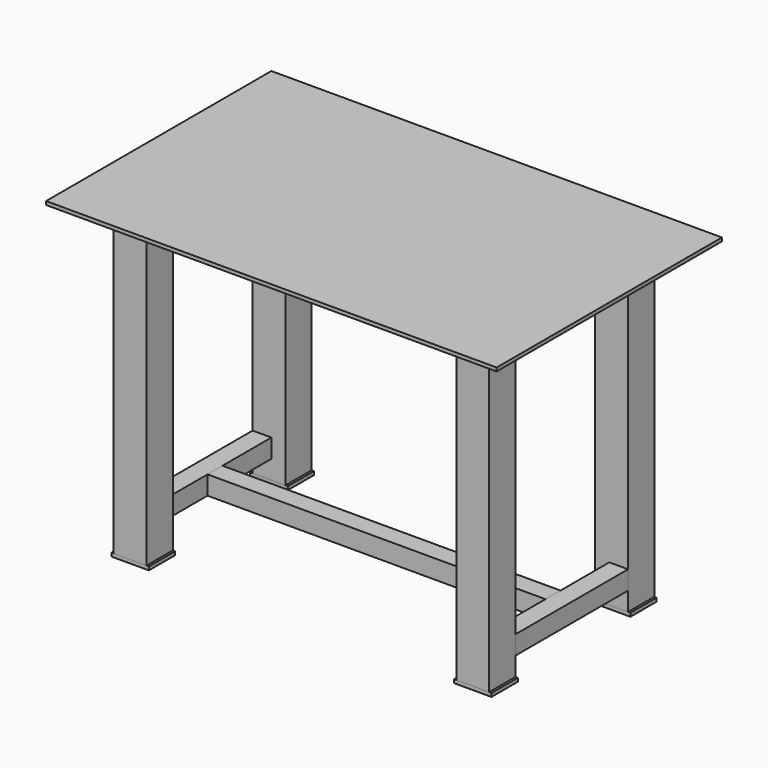
from build123d import *

# Parameters (mm, degrees)
F0_W           = 88.9
F0_H           = 88.9
F0_W_2         = 82.55
F0_H_2         = 82.55
F1_DEPTH       = 838.2
F2_W           = 50.8
F2_H           = 50.8
F2_W_2         = 46.83125
F2_H_2         = 46.83125
F3_DEPTH       = 419.1
F3_DEPTH_BACK  = 419.1
F4_W           = 50.8
F4_H           = 50.8
F4_W_2         = 46.83125
F4_H_2         = 46.83125
F5_DEPTH       = 190.5
F5_DEPTH_BACK  = 190.5
F6_W           = 50.8
F6_H           = 50.8
F6_W_2         = 46.83125
F6_H_2         = 46.83125
F7_DEPTH       = 457.2
F7_DEPTH_BACK  = 457.2
F8_W           = 1219.2
F8_H           = 762
F9_DEPTH       = 9.525
F11_W          = 101.6
F11_H          = 88.9
F12_DEPTH      = 9.525
F15_D          = 7.9375
F15_DEPTH      = 9.525
F15_TIP        = 2.3846655818
F18_W          = 50.8
F18_H          = 50.8
F18_W_2        = 46.83125
F18_H_2        = 46.83125
F19_DEPTH      = 228.6
F19_DEPTH_BACK = 228.6


# Not quite as in the source:
# - a length typed as a fraction of an inch, garbled in the dataset ("3 / 203.2 mm" for 3/8 in), is restored


with BuildPart() as f1:
    # F0 (on Top) → F1 (new body)
    with BuildSketch(Plane.XY):
        with Locations((463.55, -234.95)):
            Rectangle(F0_W, F0_H)
        with Locations((463.55, -234.95)):
            Rectangle(F0_W_2, F0_H_2, mode=Mode.SUBTRACT)
    extrude(amount=-F1_DEPTH)


with BuildPart() as f1b:
    # F0 (on Top) → F1, piece 2 (new body)
    with BuildSketch(Plane.XY):
        with Locations((463.55, 234.95)):
            Rectangle(F0_W, F0_H)
        with Locations((463.55, 234.95)):
            Rectangle(F0_W_2, F0_H_2, mode=Mode.SUBTRACT)
    extrude(amount=-F1_DEPTH)


with BuildPart() as f1c:
    # F0 (on Top) → F1, piece 3 (new body)
    with BuildSketch(Plane.XY):
        with Locations((-463.55, -234.95)):
            Rectangle(F0_W, F0_H)
        with Locations((-463.55, -234.95)):
            Rectangle(F0_W_2, F0_H_2, mode=Mode.SUBTRACT)
    extrude(amount=-F1_DEPTH)


with BuildPart() as f1d:
    # F0 (on Top) → F1, piece 4 (new body)
    with BuildSketch(Plane.XY):
        with Locations((-463.55, 234.95)):
            Rectangle(F0_W, F0_H)
        with Locations((-463.55, 234.95)):
            Rectangle(F0_W_2, F0_H_2, mode=Mode.SUBTRACT)
    extrude(amount=-F1_DEPTH)


with BuildPart() as f3:
    # F2 (on Right) → F3 (new body, two sides)
    with BuildSketch(Plane.YZ) as f3_sk:
        with Locations((-254, -25.4)):
            Rectangle(F2_W, F2_H)
        with Locations((-254, -25.4)):
            Rectangle(F2_W_2, F2_H_2, mode=Mode.SUBTRACT)
    extrude(amount=F3_DEPTH)
    extrude(f3_sk.sketch, amount=-F3_DEPTH_BACK)


with BuildPart() as f3b:
    # F2 (on Right) → F3, piece 2 (new body, two sides)
    with BuildSketch(Plane.YZ) as f3_2_sk:
        with Locations((254, -25.4)):
            Rectangle(F2_W, F2_H)
        with Locations((254, -25.4)):
            Rectangle(F2_W_2, F2_H_2, mode=Mode.SUBTRACT)
    extrude(amount=F3_DEPTH)
    extrude(f3_2_sk.sketch, amount=-F3_DEPTH_BACK)


with BuildPart() as f5:
    # F4 (on Front) → F5 (new body, two sides)
    with BuildSketch(Plane.XZ) as f5_sk:
        with Locations((-482.6, -25.4)):
            Rectangle(F4_W, F4_H)
        with Locations((-482.6, -25.4)):
            Rectangle(F4_W_2, F4_H_2, mode=Mode.SUBTRACT)
    extrude(amount=F5_DEPTH)
    extrude(f5_sk.sketch, amount=-F5_DEPTH_BACK)


with BuildPart() as f5b:
    # F4 (on Front) → F5, piece 2 (new body, two sides)
    with BuildSketch(Plane.XZ) as f5_2_sk:
        with Locations((482.6, -25.4)):
            Rectangle(F4_W, F4_H)
        with Locations((482.6, -25.4)):
            Rectangle(F4_W_2, F4_H_2, mode=Mode.SUBTRACT)
    extrude(amount=F5_DEPTH)
    extrude(f5_2_sk.sketch, amount=-F5_DEPTH_BACK)


with BuildPart() as f5c:
    # F4 (on Front) → F5, piece 3 (new body, two sides)
    with BuildSketch(Plane.XZ) as f5_3_sk:
        with Locations((-482.6, -762)):
            Rectangle(F4_W, F4_H)
        with Locations((-482.6, -762)):
            Rectangle(F4_W_2, F4_H_2, mode=Mode.SUBTRACT)
    extrude(amount=F5_DEPTH)
    extrude(f5_3_sk.sketch, amount=-F5_DEPTH_BACK)


with BuildPart() as f5d:
    # F4 (on Front) → F5, piece 4 (new body, two sides)
    with BuildSketch(Plane.XZ) as f5_4_sk:
        with Locations((482.6, -762)):
            Rectangle(F4_W, F4_H)
        with Locations((482.6, -762)):
            Rectangle(F4_W_2, F4_H_2, mode=Mode.SUBTRACT)
    extrude(amount=F5_DEPTH)
    extrude(f5_4_sk.sketch, amount=-F5_DEPTH_BACK)


with BuildPart() as f7:
    # F6 (on Right) → F7 (new body, two sides)
    with BuildSketch(Plane.YZ) as f7_sk:
        with Locations((0, -762)):
            Rectangle(F6_W, F6_H)
        with Locations((0, -762)):
            Rectangle(F6_W_2, F6_H_2, mode=Mode.SUBTRACT)
    extrude(amount=F7_DEPTH)
    extrude(f7_sk.sketch, amount=-F7_DEPTH_BACK)


with BuildPart() as f9:
    # F8 (on Top) → F9 (new body)
    with BuildSketch(Plane.XY):
        Rectangle(F8_W, F8_H)
    extrude(amount=F9_DEPTH)


with BuildPart() as f12:
    # F11 (on offset) → F12 (new body)
    with BuildSketch(Plane(origin=(0, 0, -838.2), x_dir=(1, 0, 0), z_dir=(0, 0, -1))):
        with Locations((-463.55, 234.95)):
            Rectangle(F11_W, F11_H)
    extrude(amount=F12_DEPTH)

    # F15
    with Locations(Plane(origin=(0, 0, -847.725), x_dir=(1, 0, 0), z_dir=(0, 0, -1))):
        with Locations((-500.0625, 257.175), (-500.0625, 212.725), (-427.0375, 212.725), (-427.0375, 257.175)):
            Hole(F15_D / 2, depth=F15_DEPTH)
            with Locations((0, 0, -(F15_DEPTH + F15_TIP / 2))):  # 118° drill point
                Cone(0, F15_D / 2, F15_TIP, mode=Mode.SUBTRACT)


with BuildPart() as f16_1:
    # F16: instance of F12
    add(f12.part.mirror(Plane.XZ))


with BuildPart() as f17_1:
    # F17: instance of F12
    add(f12.part.mirror(Plane.YZ))


with BuildPart() as f17_2:
    # F17: instance of F16_1
    add(f16_1.part.mirror(Plane.YZ))


with BuildPart() as f19:
    # F18 (on Front) → F19 (new body, two sides)
    with BuildSketch(Plane.XZ) as f19_sk:
        with Locations((0, -25.4)):
            Rectangle(F18_W, F18_H)
        with Locations((0, -25.4)):
            Rectangle(F18_W_2, F18_H_2, mode=Mode.SUBTRACT)
    extrude(amount=F19_DEPTH)
    extrude(f19_sk.sketch, amount=-F19_DEPTH_BACK)


solid = Compound([f1.part, f1b.part, f1c.part, f1d.part, f3.part, f3b.part, f5.part, f5b.part, f5c.part, f5d.part, f7.part, f9.part, f12.part, f16_1.part, f17_1.part, f17_2.part, f19.part])
